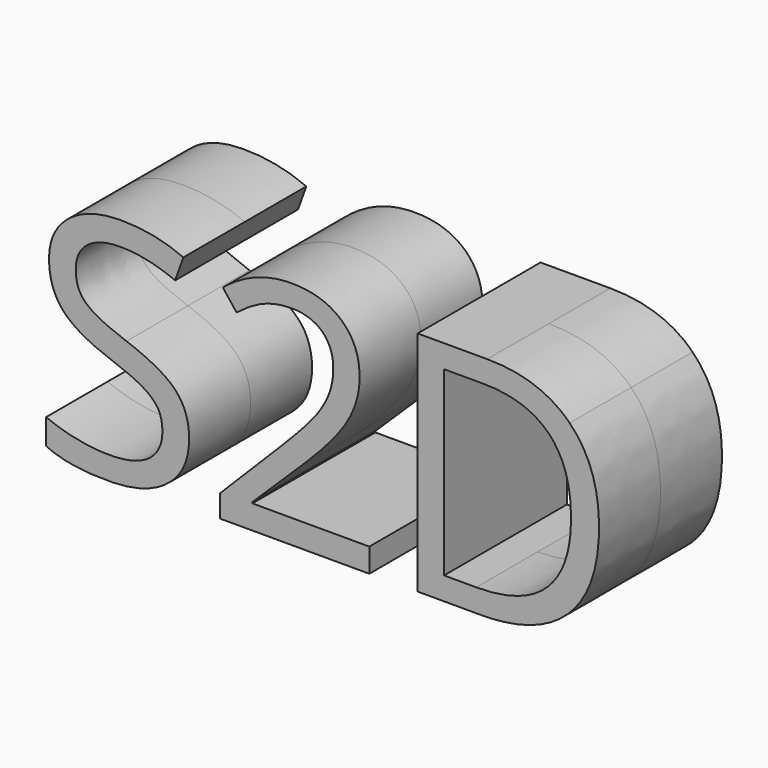
from build123d import *

# Parameters (mm, degrees)
F1_DEPTH     = 12.7
F0_TEXT_SIZE = 52.6200359066
F2_DEPTH     = 12.7


# Not quite as in the source:
# - Text() gives the source's letters only with a copy of the font that has no kerning and outlines rounded to 1/6400 em; it was checked with that copy


with BuildPart() as f1:
    # F0 (on Front) → F1 (new body, symmetric)
    with BuildSketch(Plane.XZ):
        with BuildLine():
            add(Edge.make_bspline(
                [(46.6810623863, 0.4910139833), (46.6810623863, -8.8079329871), (41.6328276915, -13.7287285324)],
                knots=[0, 0, 0, 1, 1, 1], degree=2))
            add(Edge.make_bspline(
                [(41.8260418858, 14.0612279307), (46.6810623863, 9.2062074303), (46.6810623863, 0.4910139833)],
                knots=[0, 0, 0, 1, 1, 1], degree=2))
            add(Edge.make_bspline(
                [(28.2064966547, 18.9162484312), (36.9710213854, 18.9162484312), (41.8260418858, 14.0612279307)],
                knots=[0, 0, 0, 1, 1, 1], degree=2))
            Line((28.2064966547, 18.9162484312), (16.6958638001, 18.9162484312))
            Line((16.6958638001, 18.9162484312), (16.6958638001, -18.6495240778))
            Line((16.6958638001, -18.6495240778), (27.1047646529, -18.6495240778))
            add(Edge.make_bspline(
                [(41.6328276915, -13.7287285324), (36.5845929967, -18.6495240778), (27.1047646529, -18.6495240778)],
                knots=[0, 0, 0, 1, 1, 1], degree=2))
        make_face()
        with BuildLine():
            add(Edge.make_bspline(
                [(42.0603654832, 0.3347982517), (42.0603654832, 7.6851595174), (38.3728520295, 11.4096714339)],
                knots=[0, 0, 0, 1, 1, 1], degree=2))
            add(Edge.make_bspline(
                [(38.1261956112, -11.0319516922), (42.0603654832, -7.1882225069), (42.0603654832, 0.3347982517)],
                knots=[0, 0, 0, 1, 1, 1], degree=2))
            add(Edge.make_bspline(
                [(26.3812391592, -14.8756808776), (34.1920257391, -14.8756808776), (38.1261956112, -11.0319516922)],
                knots=[0, 0, 0, 1, 1, 1], degree=2))
            Line((26.3812391592, -14.8756808776), (21.0616824043, -14.8756808776))
            Line((21.0616824043, -14.8756808776), (21.0616824043, 15.1341833504))
            Line((21.0616824043, 15.1341833504), (27.4089742355, 15.1341833504))
            add(Edge.make_bspline(
                [(38.3728520295, 11.4096714339), (34.6853385757, 15.1341833504), (27.4089742355, 15.1341833504)],
                knots=[0, 0, 0, 1, 1, 1], degree=2))
        make_face(mode=Mode.SUBTRACT)
    extrude(amount=F1_DEPTH, both=True)

    # F0 (on Front) → F2 (join, symmetric)
    with BuildSketch(Plane.XZ):
        with Locations((-47.4348049611, -18.6495240778)):
            Text('S2D', F0_TEXT_SIZE, font='Open Sans', text_align=(TextAlign.LEFT, TextAlign.BOTTOM))
    extrude(amount=F2_DEPTH, both=True)


solid = f1.part
